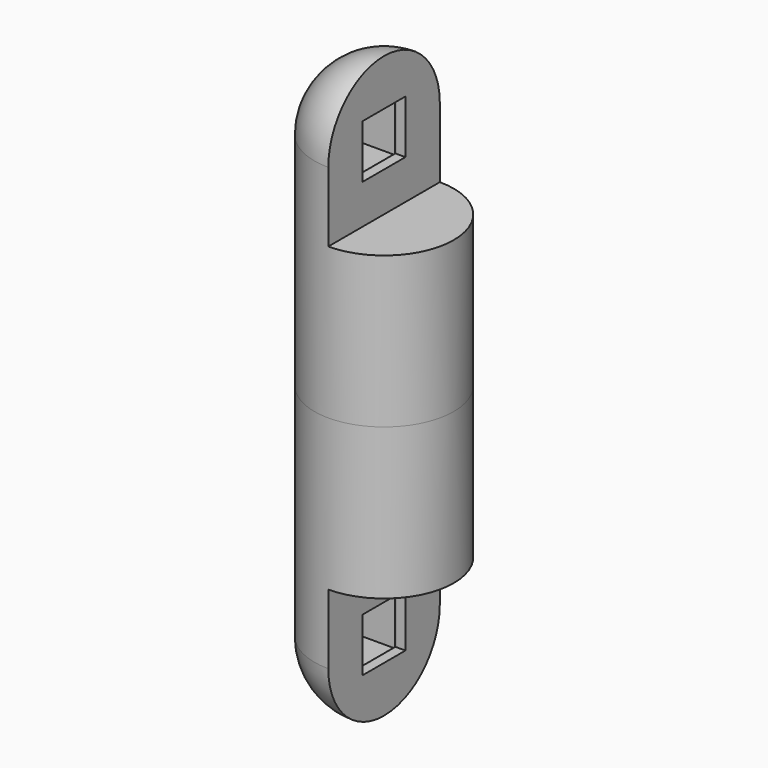
from build123d import *

# Parameters (mm, degrees)
F0_R     = 6
F1_DEPTH = 25
F2_R     = 6
F3_W     = 7.4530789975
F3_H     = 13.9023570546
F4_DEPTH = 12.5
F5_W     = 5.4
F5_H     = 5.4
F6_DEPTH = 25
F7_W     = 5.4
F7_H     = 5.4
F7_W_2   = 4.6
F7_H_2   = 4.6
F8_DEPTH = 1
F9_R     = 0.19999


# Not quite as in the source:
# - a fillet or chamfer is up to 0.001 mm smaller than in the source, because OpenCascade refuses the exact size


with BuildPart() as f1:
    # F0 (on Top) → F1 (new body)
    with BuildSketch(Plane.XY):
        Circle(F0_R)
    extrude(amount=F1_DEPTH)

    # F2
    f2_edges = [f1.edges().sort_by_distance(p)[0] for p in [
        (-6, 0, 25),
    ]]
    fillet(f2_edges, radius=F2_R)

    # F3 (on Front) → F4 (cut, symmetric)
    with BuildSketch(Plane.XZ):
        with Locations((3.7265394987, 19.9511785273)):
            Rectangle(F3_W, F3_H)
    extrude(amount=F4_DEPTH, both=True, mode=Mode.SUBTRACT)

    # F5 (on face) → F6 (cut)
    with BuildSketch(Plane.YZ):
        with Locations((0, 18.7)):
            Rectangle(F5_W, F5_H)
    extrude(amount=-F6_DEPTH, mode=Mode.SUBTRACT)

    # F7 (on face) → F8 (join)
    with BuildSketch(Plane.YZ):
        with Locations((0, 18.7)):
            Rectangle(F7_W, F7_H)
        with Locations((0, 18.7)):
            Rectangle(F7_W_2, F7_H_2, mode=Mode.SUBTRACT)
    extrude(amount=-F8_DEPTH)

    # F9 (radius 0.2 in the source; OpenCascade refuses exactly that, so slightly less here)
    f9_edges = [f1.edges().sort_by_distance(p)[0] for p in [
        (-1, 0, 16.4),
        (-1, 2.3, 18.7),
        (-1, 0, 21),
        (-1, -2.3, 18.7),
        (-1, 0, 21.4),
        (-1, -2.7, 18.7),
        (-1, 2.7, 18.7),
        (-1, 0, 16),
    ]]
    fillet(f9_edges, radius=F9_R)

    # F10: F1 across plane


with BuildPart() as f1_1:
    add(f1.part)
    add(f1.part.mirror(Plane.XY))


solid = f1_1.part
